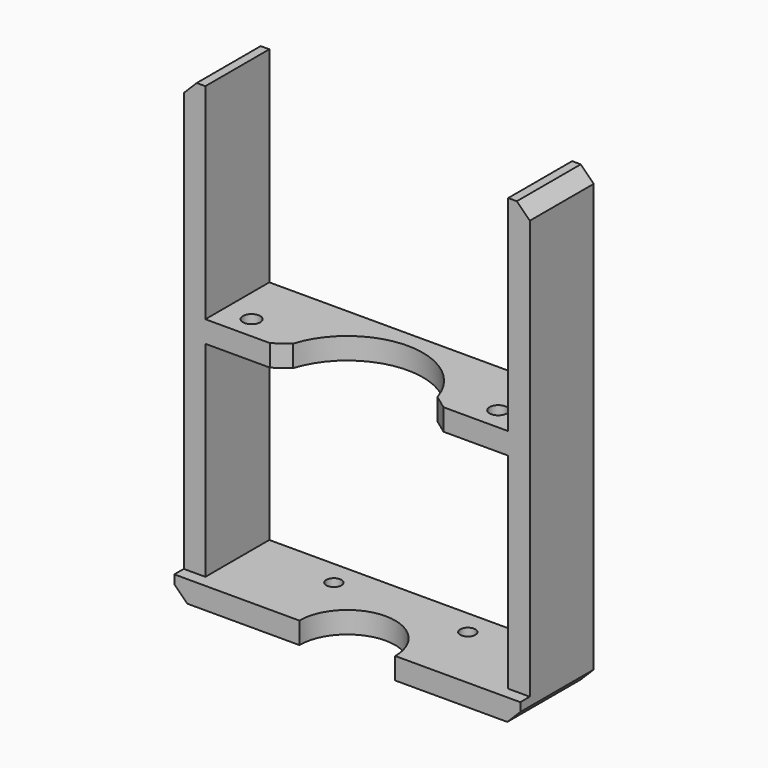
from build123d import *

# Parameters (mm, degrees)
F0_R        = 1.75
F1_DEPTH    = 5
F2_W        = 5
F2_H        = 18.5
F3_DEPTH    = 100
F4_W        = 18.5
F4_H        = 5
F5_DEPTH    = 70.1
F6_R        = 17.5
F6_R_2      = 2
F7_DEPTH    = 25
F8_SIZE     = 3
F9_T1_DEPTH = 19.3723210726


# Not quite as in the source:
# - a fillet or chamfer that OpenCascade refuses, or shapes differently, is made with other operations: its cross-section is extruded or revolved along the edge and cut away or added


with BuildPart() as f1:
    # F0 (on Top) → F1 (new body)
    with BuildSketch(Plane.XY):
        with BuildLine():
            ThreePointArc((-11.1, 0), (0, 11.1), (11.1, 0))
            Line((11.1, 0), (40.05, 0))
            Line((40.05, 0), (40.05, 21.25))
            Line((40.05, 21.25), (-40.05, 21.25))
            Line((-40.05, 21.25), (-40.05, 0))
            Line((-40.05, 0), (-11.1, 0))
        make_face()
        with Locations((-15.5, 15.5)):
            Circle(F0_R, mode=Mode.SUBTRACT)
        with Locations((15.5, 15.5)):
            Circle(F0_R, mode=Mode.SUBTRACT)
    extrude(amount=F1_DEPTH)

    # F2 (on face) → F3 (join)
    with BuildSketch(Plane.XY.offset(5)):
        with Locations((-37.55, 12)):
            Rectangle(F2_W, F2_H)
        with Locations((37.55, 12)):
            Rectangle(F2_W, F2_H)
    extrude(amount=F3_DEPTH)

    # F4 (on face) → F5 (join, through all)
    with BuildSketch(Plane(origin=(35.05, 0, 0), x_dir=(0, -1, 0), z_dir=(-1, 0, 0))):
        with Locations((-12, 55)):
            Rectangle(F4_W, F4_H)
    extrude(amount=F5_DEPTH)

    # F6 (on face) → F7 (cut)
    with BuildSketch(Plane(origin=(0, 0, 52.5), x_dir=(1, 0, 0), z_dir=(0, 0, -1))):
        Circle(F6_R)
        with Locations((-28.55, -8)):
            Circle(F6_R_2)
        with Locations((28.55, -8)):
            Circle(F6_R_2)
    extrude(amount=-F7_DEPTH, mode=Mode.SUBTRACT)

    # F8
    f8_edges = [f1.edges().sort_by_distance(p)[0] for p in [
        (-40.05, 10.625, 0),
        (40.05, 10.625, 0),
        (-40.05, 12, 105),
        (40.05, 12, 105),
    ]]
    chamfer(f8_edges, length=F8_SIZE)

    # F9: chamfer of 3 on 2 edges, made by hand

    # F9_s2 → F9_t1 (cut)
    with BuildSketch(Plane.XY.offset(45.3138394637)):
        with BuildLine():
            Line((-20.1561629778, 2.678911963), (-16.6075492446, 5.288253662))
            Line((-16.6075492446, 5.288253662), (-16.5502776109, 5.270366237))
            ThreePointArc((-16.5502776109, 5.270366237), (-16.9692117334, 4.0248544257), (-17.2233233798, 2.7405714286))
            Line((-17.2233233798, 2.7405714286), (-17.2825779327, 2.69))
            ThreePointArc((-17.2825779327, 2.69), (-18.7193704553, 2.69), (-20.1561629778, 2.618911963))
            Line((-20.1561629778, 2.618911963), (-20.1561629778, 2.678911963))
        make_face()
        with BuildLine():
            Line((20.1561629778, 2.678911963), (16.6075492446, 5.288253662))
            Line((16.6075492446, 5.288253662), (16.5502776109, 5.270366237))
            ThreePointArc((16.5502776109, 5.270366237), (16.9692117334, 4.0248544257), (17.2233233798, 2.7405714286))
            Line((17.2233233798, 2.7405714286), (17.2825779327, 2.69))
            ThreePointArc((17.2825779327, 2.69), (18.7193704553, 2.69), (20.1561629778, 2.618911963))
            Line((20.1561629778, 2.618911963), (20.1561629778, 2.678911963))
        make_face()
    extrude(amount=F9_T1_DEPTH, mode=Mode.SUBTRACT)


solid = f1.part
